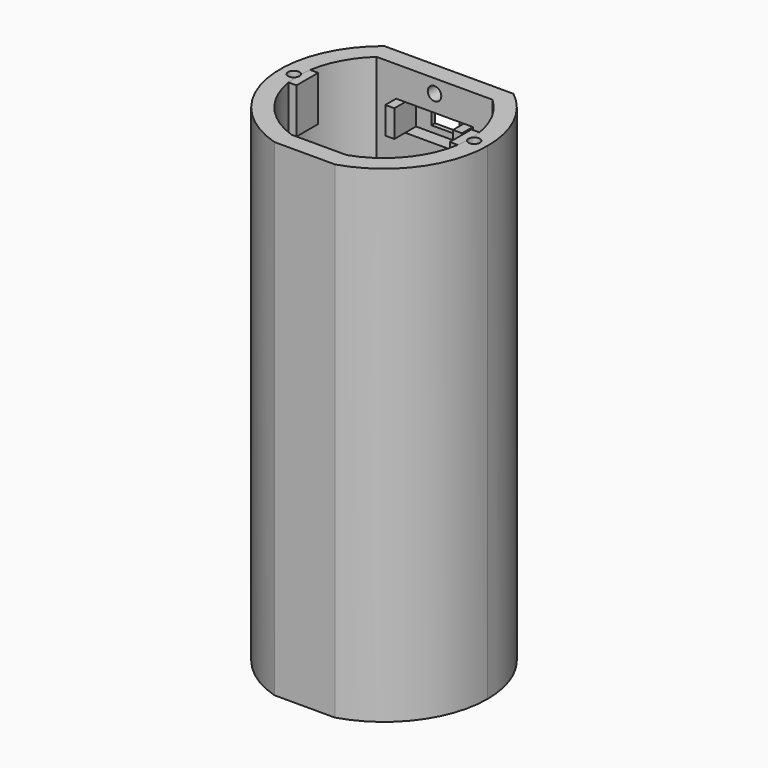
from build123d import *
from build123d import SkipClean  # not in build123d's __all__

# Parameters (mm, degrees)
F1_DEPTH  = 108
F3_DEPTH  = 105
F4_W      = 6.2
F4_H      = 3.3
F5_DEPTH  = 4
F4_R      = 3.3
F6_DEPTH  = 2.5
F8_DEPTH  = 1.5
F4_R_2    = 1.5
F9_DEPTH  = 4
F10_W     = 13
F10_H     = 6
F10_W_2   = 6.2
F10_H_2   = 3.3
F11_DEPTH = 3
F10_W_3   = 2
F12_DEPTH = 3
F14_DEPTH = 10
F15_DEPTH = 10


# Not quite as in the source:
# - a feature names something its author has since deleted; it is built from what else it names


with BuildPart() as f1:
    # F0 (on Top) → F1 (new body)
    with BuildSketch(Plane.XY):
        with BuildLine():
            ThreePointArc((6.7082039325, -22), (18.4836237038, -13.6877921805), (23, 0))
            ThreePointArc((23, 0), (20.7160551802, 9.9922498854), (14.3178210633, 18))
            Line((14.3178210633, 18), (-14.3178210633, 18))
            ThreePointArc((-14.3178210633, 18), (-22.5947655837, -4.2984378813), (-6.7082039325, -22))
            Line((-6.7082039325, -22), (6.7082039325, -22))
        make_face()
    extrude(amount=F1_DEPTH)

    # F2 (on face) → F3 (cut)
    with BuildSketch(Plane.XY.offset(108)):
        with BuildLine():
            Line((-6.0827625303, -18), (6.0827625303, -18))
            ThreePointArc((6.0827625303, -18), (18.5894391984, -3.9284539311), (12.8452325787, 14))
            Line((12.8452325787, 14), (-12.8452325787, 14))
            ThreePointArc((-12.8452325787, 14), (-18.5894391984, -3.9284539311), (-6.0827625303, -18))
        make_face()
    extrude(amount=-F3_DEPTH, mode=Mode.SUBTRACT)

    # F4 (on face) → F5 (cut)
    with BuildSketch(Plane(origin=(0, 18, 0), x_dir=(-1, 0, 0), z_dir=(0, 1, 0))):
        with Locations((0, 98.25)):
            Rectangle(F4_W, F4_H)
    extrude(amount=-F5_DEPTH, mode=Mode.SUBTRACT)

    # F4 (on face) → F6 (cut)
    with BuildSketch(Plane(origin=(0, 18, 0), x_dir=(-1, 0, 0), z_dir=(0, 1, 0))):
        with Locations((0, 89.3424802274)):
            Circle(F4_R)
    extrude(amount=-F6_DEPTH, mode=Mode.SUBTRACT)

    # F7 (on face) → F8 (cut)
    with BuildSketch(Plane(origin=(0, 15.5, 0), x_dir=(-1, 0, 0), z_dir=(0, 1, 0))):
        with BuildLine():
            ThreePointArc((3.3, 89.3424802274), (3.2424742607, 89.9559626385), (3.0719026249, 90.5480565471))
            Line((3.0719026249, 90.5480565471), (-3.0719026249, 90.5480565471))
            ThreePointArc((-3.0719026249, 90.5480565471), (-3.3, 89.3424802274), (-3.0719026249, 88.1369039076))
            Line((-3.0719026249, 88.1369039076), (3.0719026249, 88.1369039076))
            ThreePointArc((3.0719026249, 88.1369039076), (3.2424742607, 88.7289978162), (3.3, 89.3424802274))
        make_face()
    extrude(amount=-F8_DEPTH, mode=Mode.SUBTRACT)

    # F4 (on face) → F9 (cut)
    with BuildSketch(Plane(origin=(0, 18, 0), x_dir=(-1, 0, 0), z_dir=(0, 1, 0))):
        with Locations((0, 105)):
            Circle(F4_R_2)
    extrude(amount=-F9_DEPTH, mode=Mode.SUBTRACT)

    # F10 (on face) → F11 (cut)
    with BuildSketch(Plane.XZ.offset(-14)):
        with Locations((0, 98.25)):
            Rectangle(F10_W, F10_H)
        with Locations((0, 98.25)):
            Rectangle(F10_W_2, F10_H_2, mode=Mode.SUBTRACT)
    extrude(amount=-F11_DEPTH, mode=Mode.SUBTRACT)

    # F10 (on face) → F12 (join)
    with BuildSketch(Plane.XZ.offset(-14)):
        with Locations((-7.5, 98.25)):
            Rectangle(F10_W_3, F10_H)
        with Locations((7.5, 98.25)):
            Rectangle(F10_W_3, F10_H)
    extrude(amount=F12_DEPTH)

    # F13 (on face) → F14 (cut)
    with BuildSketch(Plane.XY.offset(108)):
        with BuildLine():
            ThreePointArc((21.2504766076, 0), (20.3841146719, 1.1896729952), (18.9859616706, 0.7302461521))
            ThreePointArc((18.9859616706, 0.7302461521), (18.9964900935, 0.3651905384), (19, 0))
            ThreePointArc((19, 0), (18.9964900935, -0.3651905384), (18.9859616706, -0.7302461521))
            ThreePointArc((18.9859616706, -0.7302461521), (20.3841146719, -1.1896729952), (21.2504766076, 0))
        make_face()
        with BuildLine():
            ThreePointArc((-18.9859616706, -0.7302461521), (-19, 0), (-18.9859616706, 0.7302461521))
            ThreePointArc((-18.9859616706, 0.7302461521), (-21.2504766076, 0), (-18.9859616706, -0.7302461521))
        make_face()
    extrude(amount=-F14_DEPTH, mode=Mode.SUBTRACT)

    # F13 (on face) → F15 (join)
    with BuildSketch(Plane.XY.offset(108)):
        with BuildLine():
            ThreePointArc((18.9859616706, 0.7302461521), (18.9079014817, 1.8684917869), (18.7616630393, 3))
            Line((18.7616630393, 3), (17.0004766076, 3))
            Line((17.0004766076, 3), (17.0004766076, -3))
            Line((17.0004766076, -3), (18.7616630393, -3))
            ThreePointArc((18.7616630393, -3), (18.9079014817, -1.8684917869), (18.9859616706, -0.7302461521))
            ThreePointArc((18.9859616706, -0.7302461521), (18.7504766076, 0), (18.9859616706, 0.7302461521))
        make_face()
        with BuildLine():
            Line((-17.0004766076, 3), (-18.7616630393, 3))
            ThreePointArc((-18.7616630393, 3), (-18.9079014817, 1.8684917869), (-18.9859616706, 0.7302461521))
            ThreePointArc((-18.9859616706, 0.7302461521), (-18.8108036123, 0.3836380643), (-18.7504766076, 0))
            ThreePointArc((-18.7504766076, 0), (-18.8108036123, -0.3836380643), (-18.9859616706, -0.7302461521))
            ThreePointArc((-18.9859616706, -0.7302461521), (-18.9079014817, -1.8684917869), (-18.7616630393, -3))
            Line((-18.7616630393, -3), (-17.0004766076, -3))
            Line((-17.0004766076, -3), (-17.0004766076, 3))
        make_face()
    with SkipClean():  # cleaning this boolean's faces spoils the solid; the shape is the same uncleaned
        extrude(amount=-F15_DEPTH)


solid = f1.part
